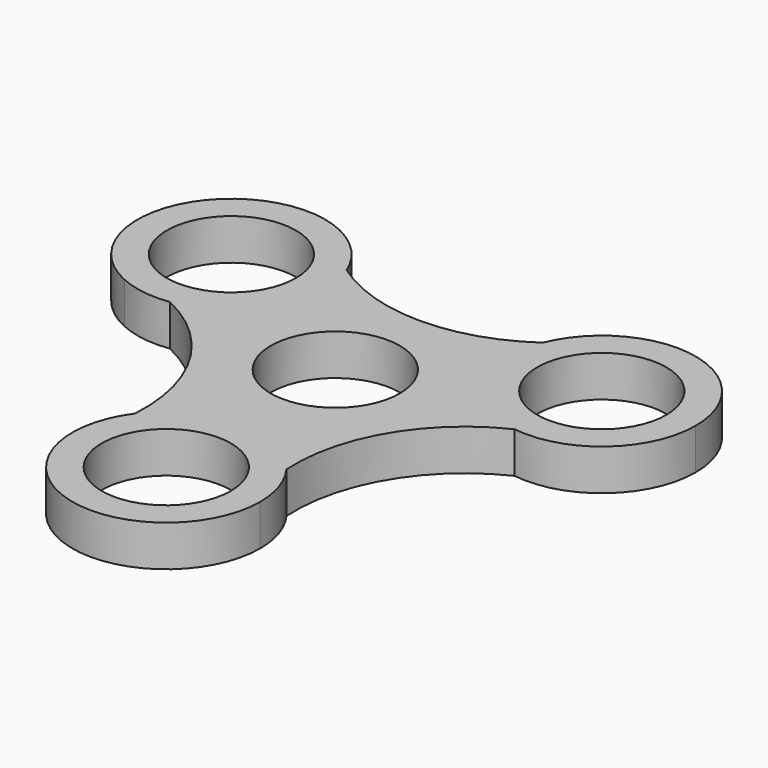
from build123d import *

# Parameters (mm, degrees)
F0_R     = 11
F1_DEPTH = 7
F2_DEPTH = 7


# Not quite as in the source:
# - a feature names something its author has since deleted; it is built from what else it names


with BuildPart() as f1:
    # F0 (on Top) → F1 (new body)
    with BuildSketch(Plane.XY):
        with BuildLine():
            ThreePointArc((29.3501442774, 1.4728811124), (17.7035935394, 9.3195381001), (16.7314646223, 23.3290753994))
            ThreePointArc((16.7314646223, 23.3290753994), (0, 18.0157402468), (-16.7314646223, 23.3290753994))
            ThreePointArc((-16.7314646223, 23.3290753994), (-15.8555966996, 20.3808641164), (-15.56, 17.3195381001))
            ThreePointArc((-15.56, 17.3195381001), (-19.4902507988, 6.8161503505), (-29.3501442774, 1.4728811124))
            ThreePointArc((-29.3501442774, 1.4728811124), (-16.8351135056, -10.0081099666), (-12.8952216464, -26.5282916699))
            ThreePointArc((-12.8952216464, -26.5282916699), (-0.0001071921, -20.0000000004), (12.8950947338, -26.5281188876))
            ThreePointArc((12.8950947338, -26.5281188876), (16.8350899961, -10.0080120701), (29.3501442774, 1.4728811124))
        make_face()
        Circle(F0_R, mode=Mode.SUBTRACT)
    extrude(amount=F1_DEPTH)

    # F0 (on Top) → F2 (join)
    with BuildSketch(Plane.XY):
        with BuildLine():
            ThreePointArc((29.3501442774, 1.4728811124), (42.0633877496, 5.2497888988), (47.56, 17.3195381001))
            ThreePointArc((47.56, 17.3195381001), (34.6213260163, 33.0239414005), (16.7314646223, 23.3290753994))
            ThreePointArc((16.7314646223, 23.3290753994), (17.7035935394, 9.3195381001), (29.3501442774, 1.4728811124))
        make_face()
        with Locations((31.56, 17.3195381001)):
            Circle(F0_R, mode=Mode.SUBTRACT)
        with BuildLine():
            ThreePointArc((-15.56, 17.3195381001), (-15.8555966996, 20.3808641164), (-16.7314646223, 23.3290753994))
            ThreePointArc((-16.7314646223, 23.3290753994), (-42.6554805123, 28.8473441446), (-38.1316823001, 2.7314267848))
            ThreePointArc((-38.1316823001, 2.7314267848), (-33.8298826127, 1.4813679746), (-29.3501442774, 1.4728811124))
            ThreePointArc((-29.3501442774, 1.4728811124), (-19.4902507988, 6.8161503505), (-15.56, 17.3195381001))
        make_face()
        with Locations((-31.56, 17.3195381001)):
            Circle(F0_R, mode=Mode.SUBTRACT)
        with BuildLine():
            ThreePointArc((16, -36), (15.2039717794, -31.0161017135), (12.8950947338, -26.5281188876))
            ThreePointArc((12.8950947338, -26.5281188876), (-0.0001071921, -20.0000000004), (-12.8952216464, -26.5282916699))
            ThreePointArc((-12.8952216464, -26.5282916699), (-4.9837964273, -51.2040051687), (16, -36))
        make_face()
        with Locations((0, -36)):
            Circle(F0_R, mode=Mode.SUBTRACT)
    extrude(amount=F2_DEPTH)


solid = f1.part
